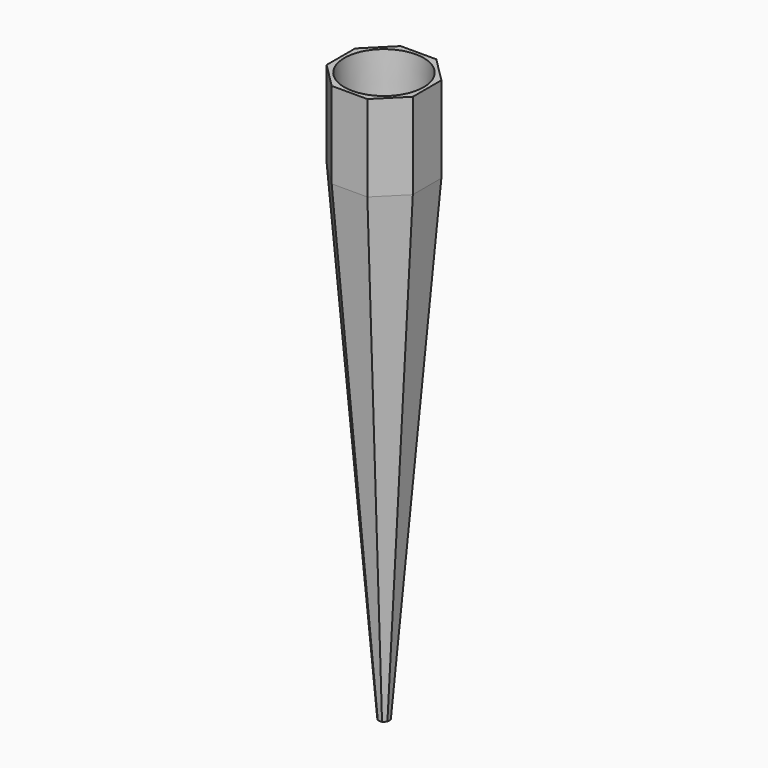
from build123d import *

# Parameters (mm, degrees)
F6_DEPTH               = 28
DRAFT_F6_DRAFTED_ANGLE = 4.5
F7_DEPTH               = 4
DRAFT_F7_DRAFTED_ANGLE = 4.5
F8_DEPTH               = 5
F9_SIZE2               = 0.19999
F9_SIZE                = 4.99999


# Not quite as in the source:
# - a fillet or chamfer is up to 0.001 mm smaller than in the source, because OpenCascade refuses the exact size
# - an extrude with a draft is written as a straight extrude whose walls are then drafted
# - a feature names something its author has since deleted; it is built from what else it names


with BuildPart() as f6:
    # F5 (on Top) → F6 (new body)
    with BuildSketch(Plane.XY):
        Polygon((-0.3827812702, -2.1), (0, -2.1), (0.3827812702, -2.1), (1.0355339059, -2.5), (2.5, -1.0355339059), (2.5, 1.0355339059), (1.0355339059, 2.5), (-1.0355339059, 2.5), (-2.5, 1.0355339059), (-2.5, -1.0355339059), (-1.0355339059, -2.5), align=None)
        with BuildLine():
            ThreePointArc((0, -2.1), (-1.4849242405, 1.4849242405), (2.1, 0))
            ThreePointArc((2.1, 0), (1.4849242405, -1.4849242405), (0, -2.1))
        make_face(mode=Mode.SUBTRACT)
        with BuildLine():
            ThreePointArc((0, -2.1), (1.4849242405, -1.4849242405), (2.1, 0))
            ThreePointArc((2.1, 0), (-1.4849242405, 1.4849242405), (0, -2.1))
        make_face()
        Polygon((0.3827812702, -2.1), (0, -2.1), (-0.3827812702, -2.1), (-1.0355339059, -2.5), (1.0355339059, -2.5), align=None)
    extrude(amount=-F6_DEPTH)

    # draft_F6_drafted
    draft_f6_drafted_walls = [f6.faces().sort_by_distance(p)[0] for p in [
        (1.767766953, -1.767766953, -18.6666666667),
        (2.5, 0, -18.6666666667),
        (1.767766953, 1.767766953, -18.6666666667),
        (0, 2.5, -18.6666666667),
        (-1.767766953, 1.767766953, -18.6666666667),
        (-2.5, 0, -18.6666666667),
        (-1.767766953, -1.767766953, -18.6666666667),
        (0, -2.5, -18.6666666667),
    ]]
    draft(draft_f6_drafted_walls, neutral_plane=Plane(origin=(0, 0, 0), x_dir=(1, 0, 0), z_dir=(0, 0, -1)), angle=DRAFT_F6_DRAFTED_ANGLE)


with BuildPart() as f7_drafted:
    # F5 (on Top) → F7 (new body)
    with BuildSketch(Plane.XY):
        with BuildLine():
            ThreePointArc((0, -2.1), (1.4849242405, -1.4849242405), (2.1, 0))
            ThreePointArc((2.1, 0), (-1.4849242405, 1.4849242405), (0, -2.1))
        make_face()
    extrude(amount=-F7_DEPTH)

    # draft_F7_drafted
    draft_f7_drafted_walls = [f7_drafted.faces().sort_by_distance(p)[0] for p in [
        (0, 2.1, -2.6666666667),
    ]]
    draft(draft_f7_drafted_walls, neutral_plane=Plane(origin=(0, 0, 0), x_dir=(1, 0, 0), z_dir=(0, 0, -1)), angle=DRAFT_F7_DRAFTED_ANGLE)


with BuildPart() as f6_1:
    add(f6.part)

    # join_F7_drafted: cut F7_drafted
    add(f7_drafted.part, mode=Mode.SUBTRACT)

    # F5 (on Top) → F8 (join)
    with BuildSketch(Plane.XY):
        Polygon((-0.3827812702, -2.1), (0, -2.1), (0.3827812702, -2.1), (1.0355339059, -2.5), (2.5, -1.0355339059), (2.5, 1.0355339059), (1.0355339059, 2.5), (-1.0355339059, 2.5), (-2.5, 1.0355339059), (-2.5, -1.0355339059), (-1.0355339059, -2.5), align=None)
        with BuildLine():
            ThreePointArc((0, -2.1), (-1.4849242405, 1.4849242405), (2.1, 0))
            ThreePointArc((2.1, 0), (1.4849242405, -1.4849242405), (0, -2.1))
        make_face(mode=Mode.SUBTRACT)
        Polygon((0.3827812702, -2.1), (0, -2.1), (-0.3827812702, -2.1), (-1.0355339059, -2.5), (1.0355339059, -2.5), align=None)
    extrude(amount=F8_DEPTH)

    # F9 (size 5 and 0.2 in the source; OpenCascade refuses exactly that, so slightly less here)
    f9_edges = [f6_1.edges().sort_by_distance(p)[0] for p in [
        (0, 2.1, 5),
    ]]
    f9_side = f6_1.faces().sort_by_distance((0, 2.1, 2.5))[0]
    chamfer(f9_edges, length=F9_SIZE, length2=F9_SIZE2, reference=f9_side)


solid = f6_1.part
